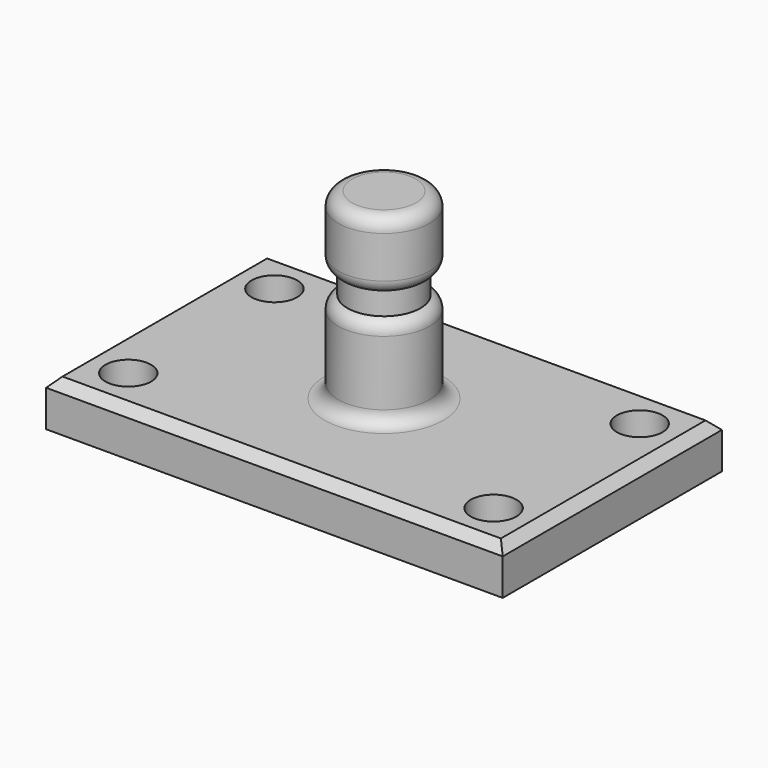
from build123d import *

# Parameters (mm, degrees)
F0_W     = 127
F0_H     = 76.2
F1_DEPTH = 12.7
F2_R     = 6.35
F3_DEPTH = 12.7
F4_W     = 12.7
F4_H     = 50.8
F6_W     = 7.1040334281
F6_H     = 6.35
F9_SIZE  = 2.54


# Not quite as in the source:
# - a fillet or chamfer that OpenCascade refuses, or shapes differently, is made with other operations: its cross-section is extruded or revolved along the edge and cut away or added


with BuildPart() as f1:
    # F0 (on Top) → F1 (new body)
    with BuildSketch(Plane.XY):
        Rectangle(F0_W, F0_H)
    extrude(amount=F1_DEPTH)

    # F2 (on face) → F3 (cut, through all)
    with BuildSketch(Plane.XY.offset(12.7)):
        with Locations((-50.8, 25.4)):
            Circle(F2_R)
        with Locations((-50.8, -25.4)):
            Circle(F2_R)
        with Locations((50.8, -25.4)):
            Circle(F2_R)
        with Locations((50.8, 25.4)):
            Circle(F2_R)
    extrude(amount=-F3_DEPTH, mode=Mode.SUBTRACT)

    # F4 (on Front) → F5 (revolve)
    with BuildSketch(Plane.XZ):
        with Locations((6.35, 38.1)):
            Rectangle(F4_W, F4_H)
    revolve(axis=Axis((0, 0, 38.1), (0, 0, 1)))

    # F6 (on Front) → F7 (revolve, cut)
    with BuildSketch(Plane.XZ):
        with Locations((13.712016714, 41.275)):
            Rectangle(F6_W, F6_H)
    revolve(axis=Axis((0, 0, 12.7), (0, 0, 1)), mode=Mode.SUBTRACT)

    # F8: fillet of radius 3.81 on 4 edges, made by hand

    # F8_s1 → F8_t2 (revolve)
    with BuildSketch(Plane.XZ):
        with BuildLine():
            ThreePointArc((16.51, 12.7), (13.8159231637, 13.8159231637), (12.7, 16.51))
            Line((12.7, 16.51), (12.7, 12.7))
            Line((12.7, 12.7), (16.51, 12.7))
        make_face()
    revolve(axis=Axis((0, 0, 12.7), (0, 0, 1)))

    # F8_s3 → F8_t4 (revolve, cut)
    with BuildSketch(Plane.XZ):
        with BuildLine():
            ThreePointArc((12.7, 34.5078975516), (12.0008519733, 36.7076020772), (10.16, 38.1))
            Line((10.16, 38.1), (12.7, 38.1))
            Line((12.7, 38.1), (12.7, 34.5078975516))
        make_face()
    revolve(axis=Axis((0, 0, 38.1), (0, 0, 1)), mode=Mode.SUBTRACT)

    # F8_s5 → F8_t6 (revolve, cut)
    with BuildSketch(Plane.XZ):
        with BuildLine():
            ThreePointArc((10.16, 44.45), (12.0008519733, 45.8423979228), (12.7, 48.0421024484))
            Line((12.7, 48.0421024484), (12.7, 44.45))
            Line((12.7, 44.45), (10.16, 44.45))
        make_face()
    revolve(axis=Axis((0, 0, 44.45), (0, 0, 1)), mode=Mode.SUBTRACT)

    # F8_s7 → F8_t8 (revolve, cut)
    with BuildSketch(Plane.XZ):
        with BuildLine():
            ThreePointArc((12.7, 59.69), (11.5840768363, 62.3840768363), (8.89, 63.5))
            Line((8.89, 63.5), (12.7, 63.5))
            Line((12.7, 63.5), (12.7, 59.69))
        make_face()
    revolve(axis=Axis((0, 0, 63.5), (0, 0, 1)), mode=Mode.SUBTRACT)

    # F9
    f9_edges = [f1.edges().sort_by_distance(p)[0] for p in [
        (0, -38.1, 12.7),
        (-63.5, 0, 12.7),
        (63.5, 0, 12.7),
        (0, 38.1, 12.7),
    ]]
    chamfer(f9_edges, length=F9_SIZE)


solid = f1.part
